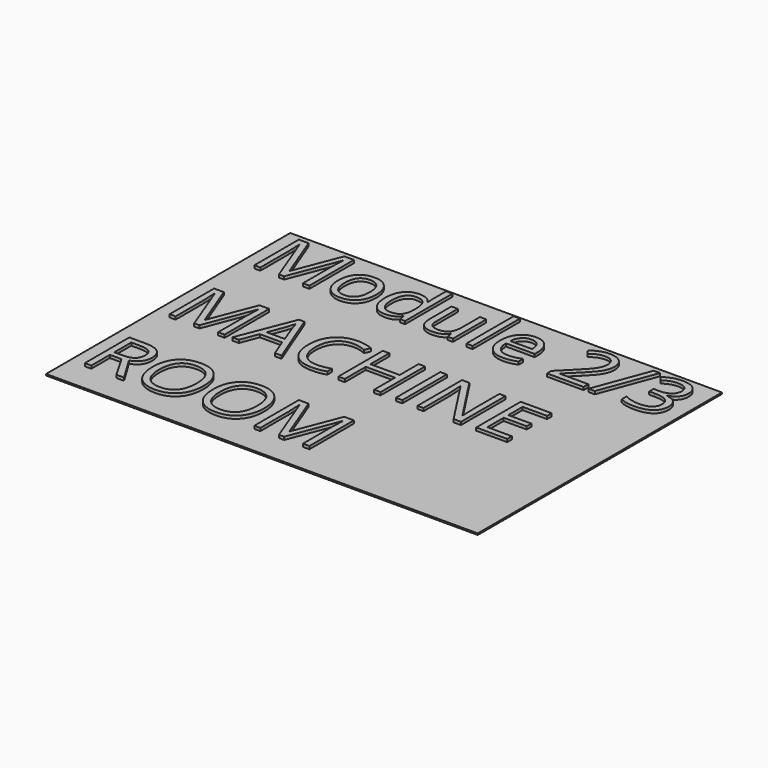
from build123d import *

# Parameters (mm, degrees)
F0_W         = 297
F0_H         = 210
F1_DEPTH     = 1
F2_TEXT_SIZE = 53.5855380197
F3_DEPTH     = 2


# Not quite as in the source:
# - Text() gives the source's letters only with a copy of the font that has no kerning and outlines rounded to 1/6400 em; it was checked with that copy


with BuildPart() as f1:
    # F0 (on Top) → F1 (new body)
    with BuildSketch(Plane.XY):
        with Locations((-47.4010080695, 34.3840229511)):
            Rectangle(F0_W, F0_H)
    extrude(amount=F1_DEPTH)

    # F2 (on face) → F3 (join)
    with BuildSketch(Plane.XY.offset(1)):
        with Locations((-190.3507038951, 94.9954763055)):
            Text('Module 2/3', F2_TEXT_SIZE, font='Open Sans', text_align=(TextAlign.LEFT, TextAlign.BOTTOM))
        with Locations((-190.3507038951, 22.1191445986)):
            Text('MACHINE', F2_TEXT_SIZE, font='Open Sans', text_align=(TextAlign.LEFT, TextAlign.BOTTOM))
        with Locations((-190.3507038951, -50.7571871082)):
            Text('ROOM', F2_TEXT_SIZE, font='Open Sans', text_align=(TextAlign.LEFT, TextAlign.BOTTOM))
    extrude(amount=F3_DEPTH)


solid = f1.part
